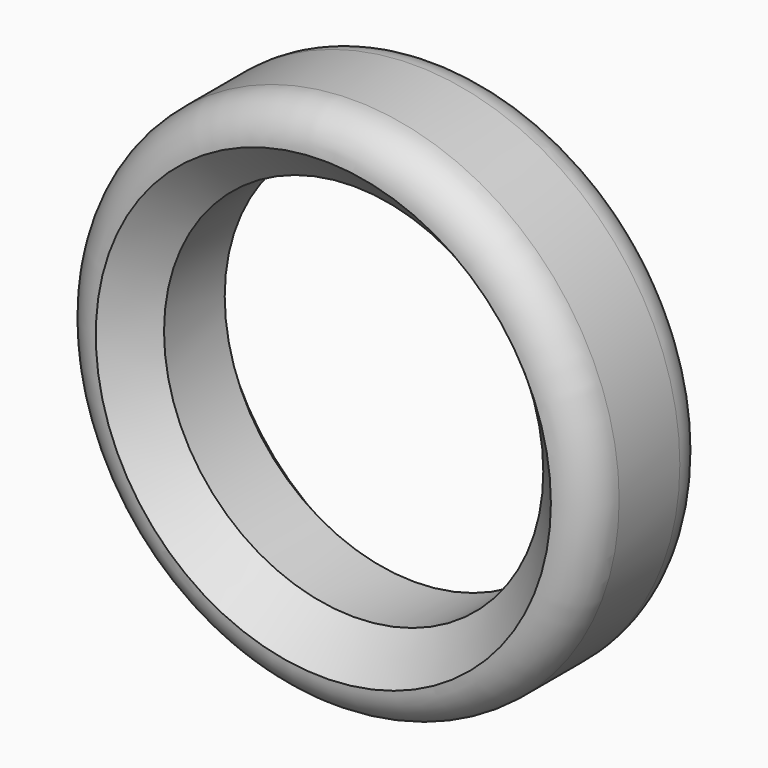
from build123d import *

# Parameters (mm, degrees)
F0_R     = 3.5
F0_R_2   = 2.5
F1_DEPTH = 2
F2_R     = 0.5
F3_SIZE  = 0.49999


# Not quite as in the source:
# - a fillet or chamfer is up to 0.001 mm smaller than in the source, because OpenCascade refuses the exact size


with BuildPart() as f1:
    # F0 (on Front) → F1 (new body)
    with BuildSketch(Plane.XZ):
        Circle(F0_R)
        Circle(F0_R_2, mode=Mode.SUBTRACT)
    extrude(amount=F1_DEPTH)

    # F2
    f2_edges = [f1.edges().sort_by_distance(p)[0] for p in [
        (-3.5, -2, 0),
        (3.5, -1, 0),
        (-3.5, 0, 0),
    ]]
    fillet(f2_edges, radius=F2_R)

    # F3 (size 0.5 in the source; OpenCascade refuses exactly that, so slightly less here)
    f3_edges = [f1.edges().sort_by_distance(p)[0] for p in [
        (-2.5, -2, 0),
        (-2.5, 0, 0),
    ]]
    chamfer(f3_edges, length=F3_SIZE)


solid = f1.part
